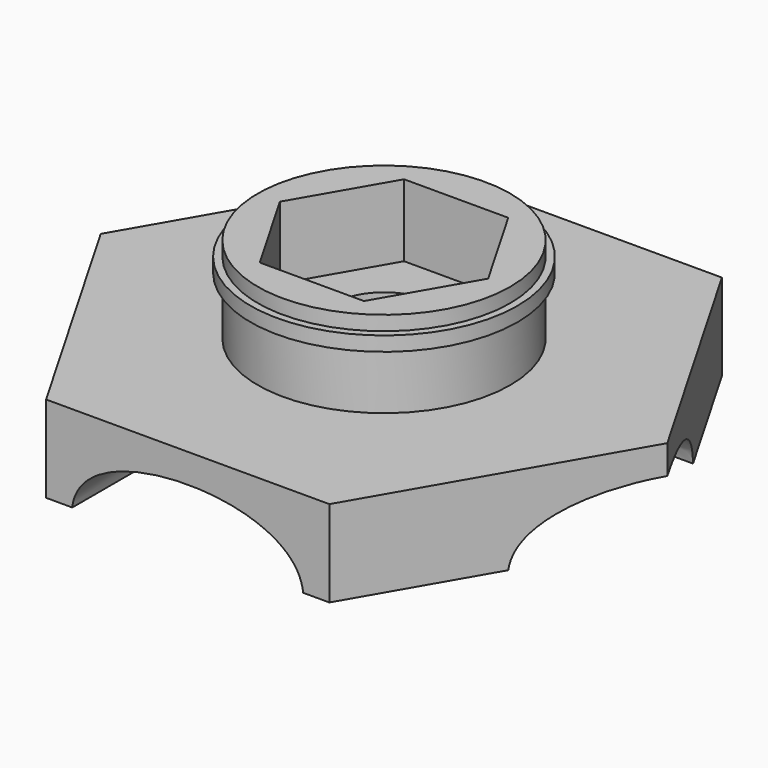
from build123d import *

# Parameters (mm, degrees)
F1_DEPTH  = 3
F2_R      = 4.375
F3_DEPTH  = 3
F4_START  = 2
F2_R_2    = 4.625
F4_DEPTH  = 0.5
F6_DEPTH  = 2.5
F7_R      = 1.75
F8_DEPTH  = 6.001
F10_START = -3.5
F9_R      = 3
F10_DEPTH = 2.5
F12_DEPTH = 12.5
F14_DEPTH = 12.5
F15_R     = 0.499


# Not quite as in the source:
# - a fillet or chamfer is up to 0.001 mm smaller than in the source, because OpenCascade refuses the exact size
# - a feature names something its author has since deleted; it is built from what else it names


with BuildPart() as f1:
    # F0 (on Top) → F1 (new body)
    with BuildSketch(Plane.XY):
        Polygon((4.9074772881, 8.5), (-4.9074772881, 8.5), (-9.8149545762, 0), (-4.9074772881, -8.5), (4.9074772881, -8.5), (9.8149545762, 0), align=None)
    extrude(amount=F1_DEPTH)

    # F2 (on face) → F3 (join)
    with BuildSketch(Plane.XY.offset(3)):
        Circle(F2_R)
    extrude(amount=F3_DEPTH)

    # F2 (on face) → F4 (join)
    with BuildSketch(Plane.XY.offset(3).offset(F4_START)):
        Circle(F2_R_2)
        Circle(F2_R, mode=Mode.SUBTRACT)
    extrude(amount=F4_DEPTH)

    # F5 (on face) → F6 (cut)
    with BuildSketch(Plane.XY.offset(6)):
        Polygon((1.8042195912, 3.125), (-1.8042195912, 3.125), (-3.6084391824, 0), (-1.8042195912, -3.125), (1.8042195912, -3.125), (3.6084391824, 0), align=None)
    extrude(amount=-F6_DEPTH, mode=Mode.SUBTRACT)

    # F7 (on face) → F8 (cut, through all)
    with BuildSketch(Plane.XY.offset(6)):
        Circle(F7_R)
    extrude(amount=-F8_DEPTH, mode=Mode.SUBTRACT)

    # F9 (on face) → F10 (cut)
    with BuildSketch(Plane.XY.offset(6).offset(F10_START)):
        Circle(F9_R)
    extrude(amount=-F10_DEPTH, mode=Mode.SUBTRACT)

    # F11 (on Front) → F12 (cut, symmetric)
    with BuildSketch(Plane.XZ):
        with BuildLine():
            add(Edge.make_bspline(
                [(-4, 0), (-3.8521862734, 1.3663038383), (0, 2.6336961617), (6.0184298072, 0.6535967597), (0, -6.4633417779), (-4.1662435338, -1.5366582221), (-4, 0)],
                knots=[0, 0, 0, 0, 0.235329262, 0.4706585239, 0.735329262, 1, 1, 1, 1], degree=3))
        make_face()
    extrude(amount=F12_DEPTH, both=True, mode=Mode.SUBTRACT)

    # F13 (on Right) → F14 (cut, symmetric)
    with BuildSketch(Plane.YZ):
        with BuildLine():
            add(Edge.make_bspline(
                [(4, 0), (3.8521862734, 1.3663038383), (0, 2.6336961617), (-6.0184298072, 0.6535967597), (0, -6.4633417779), (4.1662435338, -1.5366582221), (4, 0)],
                knots=[0, 0, 0, 0, 0.235329262, 0.4706585239, 0.735329262, 1, 1, 1, 1], degree=3))
        make_face()
    extrude(amount=F14_DEPTH, both=True, mode=Mode.SUBTRACT)

    # F15 (radius 0.5 in the source; OpenCascade refuses exactly that, so slightly less here)
    f15_edges = [f1.edges().sort_by_distance(p)[0] for p in [
        (3.238342, -3.238342, 1.190814),
        (-3.171135, 3.171135, 1.237369),
        (1.8e-05, 3, 2),
        (3.171139, 3.171139, 1.237366),
        (2.743873, 1.212915, 1.912894),
        (2.74387, -1.21292, 1.912893),
        (-3, -1.8e-05, 2),
        (-3.171104, -3.171104, 1.237389),
        (1.8e-05, -3, 2),
    ]]
    fillet(f15_edges, radius=F15_R)


solid = f1.part
